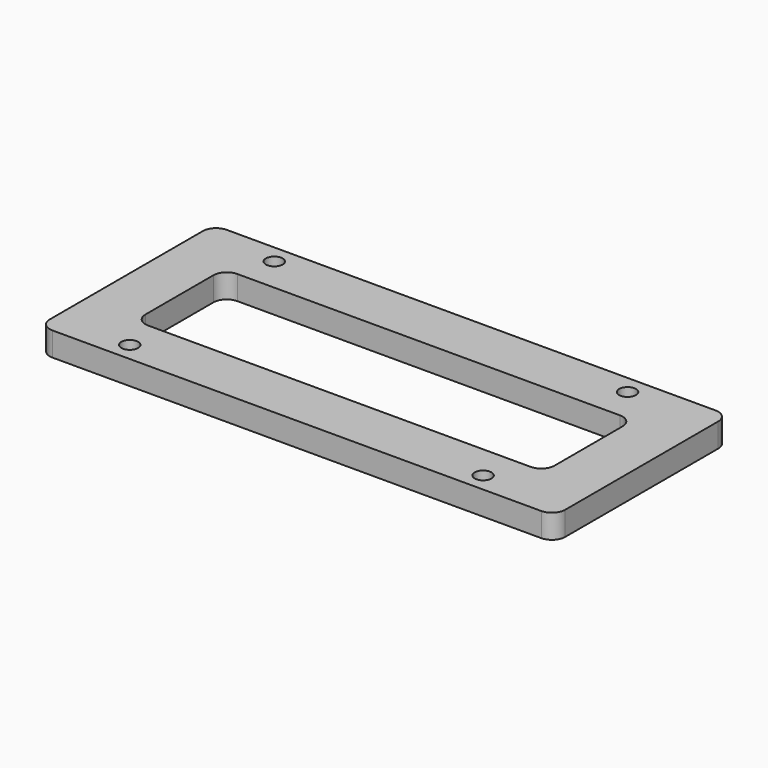
from build123d import *

# Parameters (mm, degrees)
F0_W     = 194
F0_H     = 82
F0_R     = 3.15
F0_W_2   = 154
F0_H_2   = 42
F0_R_2   = 1.75
F1_DEPTH = 9
F2_DEPTH = 6
F3_R     = 5


# Not quite as in the source:
# - a feature names something its author has since deleted; it is built from what else it names


with BuildPart() as f1:
    # F0 (on Top) → F1 (new body)
    with BuildSketch(Plane.XY):
        Rectangle(F0_W, F0_H)
        with Locations((-68.5, -34)):
            Circle(F0_R, mode=Mode.SUBTRACT)
        with Locations((64.5, -34)):
            Circle(F0_R, mode=Mode.SUBTRACT)
        with Locations((-68.5, 34)):
            Circle(F0_R, mode=Mode.SUBTRACT)
        Rectangle(F0_W_2, F0_H_2, mode=Mode.SUBTRACT)
        with Locations((64.5, 34)):
            Circle(F0_R, mode=Mode.SUBTRACT)
        with Locations((-68.5, 34)):
            Circle(F0_R)
        with Locations((-68.5, 34)):
            Circle(F0_R_2, mode=Mode.SUBTRACT)
        with Locations((-68.5, -34)):
            Circle(F0_R)
        with Locations((-68.5, -34)):
            Circle(F0_R_2, mode=Mode.SUBTRACT)
        with Locations((64.5, 34)):
            Circle(F0_R)
        with Locations((64.5, 34)):
            Circle(F0_R_2, mode=Mode.SUBTRACT)
        with Locations((64.5, -34)):
            Circle(F0_R)
        with Locations((64.5, -34)):
            Circle(F0_R_2, mode=Mode.SUBTRACT)
    extrude(amount=-F1_DEPTH)

    # F0 (on Top) → F2 (cut)
    with BuildSketch(Plane.XY):
        with Locations((-68.5, 34)):
            Circle(F0_R)
        with Locations((-68.5, 34)):
            Circle(F0_R_2, mode=Mode.SUBTRACT)
        with Locations((-68.5, -34)):
            Circle(F0_R)
        with Locations((-68.5, -34)):
            Circle(F0_R_2, mode=Mode.SUBTRACT)
        with Locations((64.5, 34)):
            Circle(F0_R)
        with Locations((64.5, 34)):
            Circle(F0_R_2, mode=Mode.SUBTRACT)
        with Locations((64.5, -34)):
            Circle(F0_R)
        with Locations((64.5, -34)):
            Circle(F0_R_2, mode=Mode.SUBTRACT)
    extrude(amount=-F2_DEPTH, mode=Mode.SUBTRACT)

    # F3
    f3_edges = [f1.edges().sort_by_distance(p)[0] for p in [
        (97, 41, -4.5),
        (-97, 41, -4.5),
        (-97, -41, -4.5),
        (97, -41, -4.5),
        (-77, 21, -4.5),
        (77, 21, -4.5),
        (77, -21, -4.5),
        (-77, -21, -4.5),
    ]]
    fillet(f3_edges, radius=F3_R)


solid = f1.part
